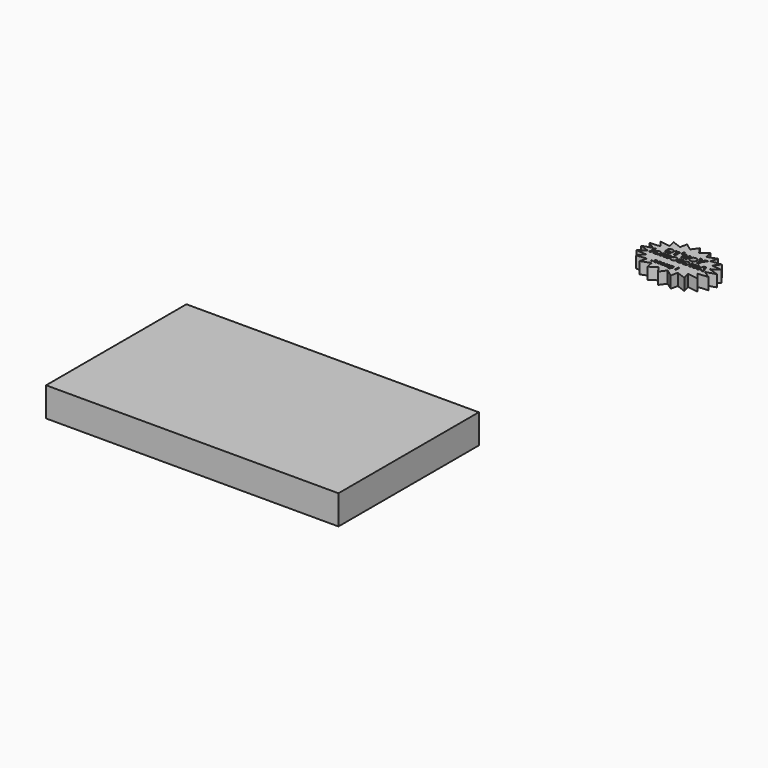
from build123d import *

# Parameters (mm, degrees)
F0_W     = 50
F0_H     = 30
F1_DEPTH = 5
F2_W     = 0.179312
F2_H     = 0.19276
F2_W_2   = 0.286899
F2_H_2   = 0.283711
F2_W_3   = 0.191765
F2_H_3   = 0.743647
F2_W_4   = 0.212485
F2_H_4   = 0.497591
F3_DEPTH = 2


# Not quite as in the source:
# - ends of sketch curves that miss each other by under 0.0002 mm in the source are joined


with BuildPart() as f1:
    # F0 (on Top) → F1 (new body)
    with BuildSketch(Plane.XY):
        with Locations((-4.7771148384, -0.2846198264)):
            Rectangle(F0_W, F0_H)
    extrude(amount=F1_DEPTH)


with BuildPart() as f3:
    # F2 (on Top) → F3 (new body)
    with BuildSketch(Plane.XY):
        Polygon((13.440635, 67.926958), (15.209908, 67.693765), (14.365041, 68.766458), (16.154706, 68.91293), (14.859046, 69.757273), (16.49392, 70.269073), (14.874297, 70.802416), (16.194345, 71.629444), (14.409299, 71.79958), (15.285305, 72.860881), (13.509569, 72.651155), (13.855785, 73.842842), (12.26318, 73.273785), (12.045715, 74.479207), (10.792136, 73.606521), (10.032278, 74.707683), (9.240434, 73.616793), (8.012563, 74.505905), (7.759965, 73.303595), (6.184273, 73.893626), (6.495648, 72.697586), (4.726375, 72.930778), (5.571243, 71.858085), (3.781577, 71.711613), (5.077236, 70.86727), (3.442363, 70.355471), (5.061986, 69.822128), (3.741938, 68.9951), (5.526984, 68.824963), (4.650977, 67.763662), (6.426714, 67.973388), (6.080498, 66.781701), (7.673103, 67.350759), (7.890568, 66.145336), (9.144147, 67.018023), (9.904005, 65.916861), (10.695849, 67.007751), (11.92372, 66.118638), (12.176318, 67.320948), (13.75201, 66.730918), align=None)
        with Locations((7.262146, 67.906265)):
            Rectangle(F2_W, F2_H, mode=Mode.SUBTRACT)
        with BuildLine():
            Line((7.542072, 68.214831), (7.542072, 68.350311))
            add(Edge.make_bspline(
                [(7.66012, 68.373721), (7.623925, 68.36874), (7.584576, 68.360937), (7.542072, 68.350311)],
                knots=[0, 0, 0, 0, 1, 1, 1, 1], degree=3))
            add(Edge.make_bspline(
                [(7.763722, 68.381192), (7.730848, 68.381192), (7.696314, 68.378702), (7.66012, 68.373721)],
                knots=[0, 0, 0, 0, 1, 1, 1, 1], degree=3))
            add(Edge.make_bspline(
                [(7.950008, 68.338357), (7.909496, 68.366913), (7.847401, 68.381192), (7.763722, 68.381192)],
                knots=[0, 0, 0, 0, 1, 1, 1, 1], degree=3))
            add(Edge.make_bspline(
                [(8.010775, 68.206861), (8.010775, 68.265968), (7.990519, 68.309799), (7.950008, 68.338357)],
                knots=[0, 0, 0, 0, 1, 1, 1, 1], degree=3))
            add(Edge.make_bspline(
                [(7.962958, 68.084331), (7.994836, 68.111228), (8.010775, 68.152071), (8.010775, 68.206861)],
                knots=[0, 0, 0, 0, 1, 1, 1, 1], degree=3))
            add(Edge.make_bspline(
                [(7.796098, 68.029043), (7.87546, 68.039005), (7.93108, 68.057434), (7.962958, 68.084331)],
                knots=[0, 0, 0, 0, 1, 1, 1, 1], degree=3))
            Line((7.796098, 68.029043), (7.764718, 68.02506))
            add(Edge.make_bspline(
                [(7.692495, 68.00663), (7.70445, 68.0146), (7.728524, 68.020743), (7.764718, 68.02506)],
                knots=[0, 0, 0, 0, 1, 1, 1, 1], degree=3))
            add(Edge.make_bspline(
                [(7.674066, 67.971266), (7.674066, 67.987205), (7.680209, 67.998993), (7.692495, 68.00663)],
                knots=[0, 0, 0, 0, 1, 1, 1, 1], degree=3))
            add(Edge.make_bspline(
                [(7.700465, 67.92843), (7.682866, 67.93806), (7.674066, 67.952339), (7.674066, 67.971266)],
                knots=[0, 0, 0, 0, 1, 1, 1, 1], degree=3))
            add(Edge.make_bspline(
                [(7.779163, 67.913986), (7.744297, 67.913986), (7.718064, 67.918801), (7.700465, 67.92843)],
                knots=[0, 0, 0, 0, 1, 1, 1, 1], degree=3))
            add(Edge.make_bspline(
                [(7.893226, 67.926936), (7.855703, 67.918303), (7.817682, 67.913986), (7.779163, 67.913986)],
                knots=[0, 0, 0, 0, 1, 1, 1, 1], degree=3))
            add(Edge.make_bspline(
                [(8.002307, 67.965787), (7.966777, 67.94852), (7.930416, 67.93557), (7.893226, 67.926936)],
                knots=[0, 0, 0, 0, 1, 1, 1, 1], degree=3))
            Line((8.002307, 67.965787), (8.002307, 67.830307))
            add(Edge.make_bspline(
                [(7.881271, 67.804406), (7.920454, 67.810051), (7.9608, 67.818685), (8.002307, 67.830307)],
                knots=[0, 0, 0, 0, 1, 1, 1, 1], degree=3))
            add(Edge.make_bspline(
                [(7.766711, 67.795441), (7.803569, 67.795441), (7.841756, 67.798429), (7.881271, 67.804406)],
                knots=[0, 0, 0, 0, 1, 1, 1, 1], degree=3))
            add(Edge.make_bspline(
                [(7.570464, 67.840269), (7.614295, 67.810383), (7.679711, 67.795441), (7.766711, 67.795441)],
                knots=[0, 0, 0, 0, 1, 1, 1, 1], degree=3))
            add(Edge.make_bspline(
                [(7.504716, 67.974255), (7.504716, 67.914816), (7.526632, 67.870154), (7.570464, 67.840269)],
                knots=[0, 0, 0, 0, 1, 1, 1, 1], degree=3))
            add(Edge.make_bspline(
                [(7.552034, 68.099275), (7.520489, 68.07271), (7.504716, 68.031037), (7.504716, 67.974255)],
                knots=[0, 0, 0, 0, 1, 1, 1, 1], degree=3))
            add(Edge.make_bspline(
                [(7.736327, 68.156555), (7.645011, 68.144933), (7.58358, 68.12584), (7.552034, 68.099275)],
                knots=[0, 0, 0, 0, 1, 1, 1, 1], degree=3))
            Line((7.736327, 68.156555), (7.767707, 68.161037))
            add(Edge.make_bspline(
                [(7.834949, 68.177973), (7.822331, 68.170335), (7.799917, 68.16469), (7.767707, 68.161037)],
                knots=[0, 0, 0, 0, 1, 1, 1, 1], degree=3))
            add(Edge.make_bspline(
                [(7.853378, 68.210846), (7.853378, 68.196568), (7.847235, 68.18561), (7.834949, 68.177973)],
                knots=[0, 0, 0, 0, 1, 1, 1, 1], degree=3))
            add(Edge.make_bspline(
                [(7.828972, 68.249697), (7.845243, 68.241396), (7.853378, 68.228446), (7.853378, 68.210846)],
                knots=[0, 0, 0, 0, 1, 1, 1, 1], degree=3))
            add(Edge.make_bspline(
                [(7.753262, 68.262648), (7.787132, 68.262648), (7.812369, 68.258331), (7.828972, 68.249697)],
                knots=[0, 0, 0, 0, 1, 1, 1, 1], degree=3))
            add(Edge.make_bspline(
                [(7.652648, 68.250693), (7.688179, 68.258663), (7.721717, 68.262648), (7.753262, 68.262648)],
                knots=[0, 0, 0, 0, 1, 1, 1, 1], degree=3))
            add(Edge.make_bspline(
                [(7.542072, 68.214831), (7.580259, 68.23077), (7.617118, 68.242724), (7.652648, 68.250693)],
                knots=[0, 0, 0, 0, 1, 1, 1, 1], degree=3))
        make_face(mode=Mode.SUBTRACT)
        with BuildLine():
            Line((8.149742, 68.214831), (8.149742, 68.350311))
            add(Edge.make_bspline(
                [(8.267789, 68.373721), (8.231594, 68.36874), (8.192245, 68.360937), (8.149742, 68.350311)],
                knots=[0, 0, 0, 0, 1, 1, 1, 1], degree=3))
            add(Edge.make_bspline(
                [(8.371391, 68.381192), (8.338517, 68.381192), (8.303983, 68.378702), (8.267789, 68.373721)],
                knots=[0, 0, 0, 0, 1, 1, 1, 1], degree=3))
            add(Edge.make_bspline(
                [(8.557677, 68.338357), (8.517165, 68.366913), (8.45507, 68.381192), (8.371391, 68.381192)],
                knots=[0, 0, 0, 0, 1, 1, 1, 1], degree=3))
            add(Edge.make_bspline(
                [(8.618444, 68.206861), (8.618444, 68.265968), (8.598188, 68.309799), (8.557677, 68.338357)],
                knots=[0, 0, 0, 0, 1, 1, 1, 1], degree=3))
            add(Edge.make_bspline(
                [(8.570627, 68.084331), (8.602505, 68.111228), (8.618444, 68.152071), (8.618444, 68.206861)],
                knots=[0, 0, 0, 0, 1, 1, 1, 1], degree=3))
            add(Edge.make_bspline(
                [(8.403767, 68.029043), (8.483129, 68.039005), (8.538749, 68.057434), (8.570627, 68.084331)],
                knots=[0, 0, 0, 0, 1, 1, 1, 1], degree=3))
            Line((8.403767, 68.029043), (8.372387, 68.02506))
            add(Edge.make_bspline(
                [(8.300164, 68.00663), (8.312119, 68.0146), (8.336193, 68.020743), (8.372387, 68.02506)],
                knots=[0, 0, 0, 0, 1, 1, 1, 1], degree=3))
            add(Edge.make_bspline(
                [(8.281735, 67.971266), (8.281735, 67.987205), (8.287878, 67.998993), (8.300164, 68.00663)],
                knots=[0, 0, 0, 0, 1, 1, 1, 1], degree=3))
            add(Edge.make_bspline(
                [(8.308134, 67.92843), (8.290535, 67.93806), (8.281735, 67.952339), (8.281735, 67.971266)],
                knots=[0, 0, 0, 0, 1, 1, 1, 1], degree=3))
            add(Edge.make_bspline(
                [(8.386832, 67.913986), (8.351966, 67.913986), (8.325733, 67.918801), (8.308134, 67.92843)],
                knots=[0, 0, 0, 0, 1, 1, 1, 1], degree=3))
            add(Edge.make_bspline(
                [(8.500894, 67.926936), (8.463372, 67.918303), (8.425351, 67.913986), (8.386832, 67.913986)],
                knots=[0, 0, 0, 0, 1, 1, 1, 1], degree=3))
            add(Edge.make_bspline(
                [(8.609976, 67.965787), (8.574446, 67.94852), (8.538085, 67.93557), (8.500894, 67.926936)],
                knots=[0, 0, 0, 0, 1, 1, 1, 1], degree=3))
            Line((8.609976, 67.965787), (8.609976, 67.830307))
            add(Edge.make_bspline(
                [(8.48894, 67.804406), (8.528123, 67.810051), (8.568469, 67.818685), (8.609976, 67.830307)],
                knots=[0, 0, 0, 0, 1, 1, 1, 1], degree=3))
            add(Edge.make_bspline(
                [(8.37438, 67.795441), (8.411238, 67.795441), (8.449425, 67.798429), (8.48894, 67.804406)],
                knots=[0, 0, 0, 0, 1, 1, 1, 1], degree=3))
            add(Edge.make_bspline(
                [(8.178133, 67.840269), (8.221964, 67.810383), (8.28738, 67.795441), (8.37438, 67.795441)],
                knots=[0, 0, 0, 0, 1, 1, 1, 1], degree=3))
            add(Edge.make_bspline(
                [(8.112385, 67.974255), (8.112385, 67.914816), (8.134301, 67.870154), (8.178133, 67.840269)],
                knots=[0, 0, 0, 0, 1, 1, 1, 1], degree=3))
            add(Edge.make_bspline(
                [(8.159703, 68.099275), (8.128158, 68.07271), (8.112385, 68.031037), (8.112385, 67.974255)],
                knots=[0, 0, 0, 0, 1, 1, 1, 1], degree=3))
            add(Edge.make_bspline(
                [(8.343996, 68.156555), (8.25268, 68.144933), (8.191249, 68.12584), (8.159703, 68.099275)],
                knots=[0, 0, 0, 0, 1, 1, 1, 1], degree=3))
            Line((8.343996, 68.156555), (8.375376, 68.161037))
            add(Edge.make_bspline(
                [(8.442618, 68.177973), (8.43, 68.170335), (8.407586, 68.16469), (8.375376, 68.161037)],
                knots=[0, 0, 0, 0, 1, 1, 1, 1], degree=3))
            add(Edge.make_bspline(
                [(8.461047, 68.210846), (8.461047, 68.196568), (8.454904, 68.18561), (8.442618, 68.177973)],
                knots=[0, 0, 0, 0, 1, 1, 1, 1], degree=3))
            add(Edge.make_bspline(
                [(8.436641, 68.249697), (8.452912, 68.241396), (8.461047, 68.228446), (8.461047, 68.210846)],
                knots=[0, 0, 0, 0, 1, 1, 1, 1], degree=3))
            add(Edge.make_bspline(
                [(8.360931, 68.262648), (8.394801, 68.262648), (8.420038, 68.258331), (8.436641, 68.249697)],
                knots=[0, 0, 0, 0, 1, 1, 1, 1], degree=3))
            add(Edge.make_bspline(
                [(8.260317, 68.250693), (8.295848, 68.258663), (8.329386, 68.262648), (8.360931, 68.262648)],
                knots=[0, 0, 0, 0, 1, 1, 1, 1], degree=3))
            add(Edge.make_bspline(
                [(8.149742, 68.214831), (8.187928, 68.23077), (8.224787, 68.242724), (8.260317, 68.250693)],
                knots=[0, 0, 0, 0, 1, 1, 1, 1], degree=3))
        make_face(mode=Mode.SUBTRACT)
        with BuildLine():
            Line((8.720054, 68.039503), (8.720054, 68.090309))
            add(Edge.make_bspline(
                [(8.79925, 68.301996), (8.746453, 68.249199), (8.720054, 68.178636), (8.720054, 68.090309)],
                knots=[0, 0, 0, 0, 1, 1, 1, 1], degree=3))
            add(Edge.make_bspline(
                [(9.009444, 68.381193), (8.92178, 68.381193), (8.851715, 68.354794), (8.79925, 68.301996)],
                knots=[0, 0, 0, 0, 1, 1, 1, 1], degree=3))
            add(Edge.make_bspline(
                [(9.236572, 68.302993), (9.181451, 68.355126), (9.105741, 68.381193), (9.009444, 68.381193)],
                knots=[0, 0, 0, 0, 1, 1, 1, 1], degree=3))
            add(Edge.make_bspline(
                [(9.318757, 68.088316), (9.318757, 68.1793), (9.291362, 68.250859), (9.236572, 68.302993)],
                knots=[0, 0, 0, 0, 1, 1, 1, 1], degree=3))
            add(Edge.make_bspline(
                [(9.235078, 67.872146), (9.290864, 67.923615), (9.318757, 67.995672), (9.318757, 68.088316)],
                knots=[0, 0, 0, 0, 1, 1, 1, 1], degree=3))
            add(Edge.make_bspline(
                [(8.999482, 67.79544), (9.100428, 67.79544), (9.17896, 67.821008), (9.235078, 67.872146)],
                knots=[0, 0, 0, 0, 1, 1, 1, 1], degree=3))
            add(Edge.make_bspline(
                [(8.872967, 67.807892), (8.915139, 67.79959), (8.95731, 67.79544), (8.999482, 67.79544)],
                knots=[0, 0, 0, 0, 1, 1, 1, 1], degree=3))
            add(Edge.make_bspline(
                [(8.746453, 67.843755), (8.788624, 67.827816), (8.830796, 67.815861), (8.872967, 67.807892)],
                knots=[0, 0, 0, 0, 1, 1, 1, 1], degree=3))
            Line((8.746453, 67.843755), (8.746453, 67.981227))
            add(Edge.make_bspline(
                [(8.867986, 67.930422), (8.828471, 67.941712), (8.78796, 67.958647), (8.746453, 67.981227)],
                knots=[0, 0, 0, 0, 1, 1, 1, 1], degree=3))
            add(Edge.make_bspline(
                [(8.983045, 67.913985), (8.945522, 67.913985), (8.907169, 67.919464), (8.867986, 67.930422)],
                knots=[0, 0, 0, 0, 1, 1, 1, 1], degree=3))
            add(Edge.make_bspline(
                [(9.091629, 67.945365), (9.065728, 67.924445), (9.029533, 67.913985), (8.983045, 67.913985)],
                knots=[0, 0, 0, 0, 1, 1, 1, 1], degree=3))
            add(Edge.make_bspline(
                [(9.136955, 68.039503), (9.132638, 67.997664), (9.117529, 67.966285), (9.091629, 67.945365)],
                knots=[0, 0, 0, 0, 1, 1, 1, 1], degree=3))
            Line((9.136955, 68.039503), (8.720054, 68.039503))
        make_face(mode=Mode.SUBTRACT)
        with BuildLine():
            Line((10.010105, 68.367745), (10.010105, 68.027051))
            add(Edge.make_bspline(
                [(9.9598, 67.854712), (9.993338, 67.894228), (10.010107, 67.951674), (10.010105, 68.027051)],
                knots=[0, 0, 0, 0, 1, 1, 1, 1], degree=3))
            add(Edge.make_bspline(
                [(9.812365, 67.79544), (9.876785, 67.79544), (9.92593, 67.815197), (9.9598, 67.854712)],
                knots=[0, 0, 0, 0, 1, 1, 1, 1], degree=3))
            add(Edge.make_bspline(
                [(9.713245, 67.818352), (9.743131, 67.803077), (9.776171, 67.79544), (9.812365, 67.79544)],
                knots=[0, 0, 0, 0, 1, 1, 1, 1], degree=3))
            add(Edge.make_bspline(
                [(9.627574, 67.890575), (9.654471, 67.858033), (9.683028, 67.833959), (9.713245, 67.818352)],
                knots=[0, 0, 0, 0, 1, 1, 1, 1], degree=3))
            Line((9.627574, 67.890575), (9.627574, 67.809885))
            Line((9.627574, 67.809885), (9.449258, 67.809885))
            Line((9.449258, 67.809885), (9.449258, 68.367745))
            Line((9.449258, 68.367745), (9.627574, 68.367745))
            Line((9.627574, 68.367745), (9.627574, 68.092301))
            add(Edge.make_bspline(
                [(9.659452, 67.973258), (9.6382, 68.001815), (9.627574, 68.041496), (9.627574, 68.092301)],
                knots=[0, 0, 0, 0, 1, 1, 1, 1], degree=3))
            add(Edge.make_bspline(
                [(9.747116, 67.930422), (9.709925, 67.930422), (9.680704, 67.944701), (9.659452, 67.973258)],
                knots=[0, 0, 0, 0, 1, 1, 1, 1], degree=3))
            add(Edge.make_bspline(
                [(9.787959, 67.939886), (9.776005, 67.933577), (9.76239, 67.930422), (9.747116, 67.930422)],
                knots=[0, 0, 0, 0, 1, 1, 1, 1], degree=3))
            add(Edge.make_bspline(
                [(9.81635, 67.966783), (9.809045, 67.955161), (9.799581, 67.946195), (9.787959, 67.939886)],
                knots=[0, 0, 0, 0, 1, 1, 1, 1], degree=3))
            add(Edge.make_bspline(
                [(9.828304, 68.009618), (9.82598, 67.990027), (9.821995, 67.975748), (9.81635, 67.966783)],
                knots=[0, 0, 0, 0, 1, 1, 1, 1], degree=3))
            add(Edge.make_bspline(
                [(9.831791, 68.106746), (9.831791, 68.061918), (9.830629, 68.029542), (9.828304, 68.009618)],
                knots=[0, 0, 0, 0, 1, 1, 1, 1], degree=3))
            add(Edge.make_bspline(
                [(9.831292, 68.197896), (9.831624, 68.152404), (9.831791, 68.122021), (9.831791, 68.106746)],
                knots=[0, 0, 0, 0, 1, 1, 1, 1], degree=3))
            add(Edge.make_bspline(
                [(9.830793, 68.311959), (9.830793, 68.281741), (9.830959, 68.24372), (9.831292, 68.197896)],
                knots=[0, 0, 0, 0, 1, 1, 1, 1], degree=3))
            Line((9.830793, 68.311959), (9.830793, 68.367745))
            Line((9.830793, 68.367745), (10.010105, 68.367745))
        make_face(mode=Mode.SUBTRACT)
        with Locations((5.4750865, 69.8638915)):
            Rectangle(F2_W_2, F2_H_2, mode=Mode.SUBTRACT)
        with BuildLine():
            Line((5.925359, 70.089427), (5.925359, 70.170715))
            add(Edge.make_bspline(
                [(6.052073, 70.509416), (5.967597, 70.42494), (5.925359, 70.31204), (5.925359, 70.170715)],
                knots=[0, 0, 0, 0, 1, 1, 1, 1], degree=3))
            add(Edge.make_bspline(
                [(6.388383, 70.63613), (6.248121, 70.63613), (6.136018, 70.593892), (6.052073, 70.509416)],
                knots=[0, 0, 0, 0, 1, 1, 1, 1], degree=3))
            add(Edge.make_bspline(
                [(6.751789, 70.51101), (6.663594, 70.594423), (6.542459, 70.63613), (6.388383, 70.63613)],
                knots=[0, 0, 0, 0, 1, 1, 1, 1], degree=3))
            add(Edge.make_bspline(
                [(6.883285, 70.167527), (6.883285, 70.313102), (6.839453, 70.427596), (6.751789, 70.51101)],
                knots=[0, 0, 0, 0, 1, 1, 1, 1], degree=3))
            add(Edge.make_bspline(
                [(6.749398, 69.821654), (6.838656, 69.904005), (6.883285, 70.019296), (6.883285, 70.167527)],
                knots=[0, 0, 0, 0, 1, 1, 1, 1], degree=3))
            add(Edge.make_bspline(
                [(6.372444, 69.698925), (6.533958, 69.698925), (6.659609, 69.739835), (6.749398, 69.821654)],
                knots=[0, 0, 0, 0, 1, 1, 1, 1], degree=3))
            add(Edge.make_bspline(
                [(6.170021, 69.718848), (6.237495, 69.705566), (6.30497, 69.698925), (6.372444, 69.698925)],
                knots=[0, 0, 0, 0, 1, 1, 1, 1], degree=3))
            add(Edge.make_bspline(
                [(5.967597, 69.776228), (6.035072, 69.750726), (6.102546, 69.731599), (6.170021, 69.718848)],
                knots=[0, 0, 0, 0, 1, 1, 1, 1], degree=3))
            Line((5.967597, 69.776228), (5.967597, 69.996184))
            add(Edge.make_bspline(
                [(6.162051, 69.914896), (6.098827, 69.93296), (6.034009, 69.960056), (5.967597, 69.996184)],
                knots=[0, 0, 0, 0, 1, 1, 1, 1], degree=3))
            add(Edge.make_bspline(
                [(6.346145, 69.888597), (6.286109, 69.888597), (6.224744, 69.897363), (6.162051, 69.914896)],
                knots=[0, 0, 0, 0, 1, 1, 1, 1], degree=3))
            add(Edge.make_bspline(
                [(6.519879, 69.938804), (6.478438, 69.905333), (6.420526, 69.888597), (6.346145, 69.888597)],
                knots=[0, 0, 0, 0, 1, 1, 1, 1], degree=3))
            add(Edge.make_bspline(
                [(6.592401, 70.089427), (6.585494, 70.022483), (6.56132, 69.972276), (6.519879, 69.938804)],
                knots=[0, 0, 0, 0, 1, 1, 1, 1], degree=3))
            Line((6.592401, 70.089427), (5.925359, 70.089427))
        make_face(mode=Mode.SUBTRACT)
        with BuildLine():
            add(Edge.make_bspline(
                [(7.691385, 70.466381), (7.655257, 70.521636), (7.612487, 70.563608), (7.563077, 70.592298)],
                knots=[0, 0, 0, 0, 1, 1, 1, 1], degree=3))
            add(Edge.make_bspline(
                [(7.798972, 70.591501), (7.751687, 70.561748), (7.715825, 70.520042), (7.691385, 70.466381)],
                knots=[0, 0, 0, 0, 1, 1, 1, 1], degree=3))
            add(Edge.make_bspline(
                [(7.962346, 70.63613), (7.900716, 70.63613), (7.846258, 70.621253), (7.798972, 70.591501)],
                knots=[0, 0, 0, 0, 1, 1, 1, 1], degree=3))
            add(Edge.make_bspline(
                [(8.112968, 70.597876), (8.067277, 70.623379), (8.017069, 70.63613), (7.962346, 70.63613)],
                knots=[0, 0, 0, 0, 1, 1, 1, 1], degree=3))
            add(Edge.make_bspline(
                [(8.233306, 70.483914), (8.198241, 70.534387), (8.158128, 70.572374), (8.112968, 70.597876)],
                knots=[0, 0, 0, 0, 1, 1, 1, 1], degree=3))
            Line((8.233306, 70.483914), (8.233306, 70.614612))
            Line((8.233306, 70.614612), (8.520206, 70.614612))
            Line((8.520206, 70.614612), (8.520206, 69.722036))
            Line((8.520206, 69.722036), (8.233306, 69.722036))
            Line((8.233306, 69.722036), (8.233306, 70.161151))
            add(Edge.make_bspline(
                [(8.188678, 70.353215), (8.21843, 70.308586), (8.233306, 70.244565), (8.233306, 70.161151)],
                knots=[0, 0, 0, 0, 1, 1, 1, 1], degree=3))
            add(Edge.make_bspline(
                [(8.061964, 70.420955), (8.116687, 70.420955), (8.158925, 70.398375), (8.188678, 70.353215)],
                knots=[0, 0, 0, 0, 1, 1, 1, 1], degree=3))
            add(Edge.make_bspline(
                [(7.971112, 70.37792), (7.988114, 70.40661), (8.018397, 70.420955), (8.061964, 70.420955)],
                knots=[0, 0, 0, 0, 1, 1, 1, 1], degree=3))
            add(Edge.make_bspline(
                [(7.94561, 70.187451), (7.94561, 70.286272), (7.954111, 70.349761), (7.971112, 70.37792)],
                knots=[0, 0, 0, 0, 1, 1, 1, 1], degree=3))
            Line((7.94561, 70.187451), (7.94561, 69.722036))
            Line((7.94561, 69.722036), (7.658711, 69.722036))
            Line((7.658711, 69.722036), (7.658711, 70.160355))
            add(Edge.make_bspline(
                [(7.613285, 70.354012), (7.642506, 70.309383), (7.657648, 70.244831), (7.658711, 70.160355)],
                knots=[0, 0, 0, 0, 1, 1, 1, 1], degree=3))
            add(Edge.make_bspline(
                [(7.487368, 70.420955), (7.54156, 70.420955), (7.583532, 70.398641), (7.613285, 70.354012)],
                knots=[0, 0, 0, 0, 1, 1, 1, 1], degree=3))
            add(Edge.make_bspline(
                [(7.397313, 70.37792), (7.415909, 70.40661), (7.445927, 70.420955), (7.487368, 70.420955)],
                knots=[0, 0, 0, 0, 1, 1, 1, 1], degree=3))
            add(Edge.make_bspline(
                [(7.36942, 70.240846), (7.36942, 70.30407), (7.378718, 70.349761), (7.397313, 70.37792)],
                knots=[0, 0, 0, 0, 1, 1, 1, 1], degree=3))
            add(Edge.make_bspline(
                [(7.370217, 70.208968), (7.369686, 70.216406), (7.36942, 70.227032), (7.36942, 70.240846)],
                knots=[0, 0, 0, 0, 1, 1, 1, 1], degree=3))
            add(Edge.make_bspline(
                [(7.371014, 70.187451), (7.370482, 70.194358), (7.370217, 70.20153), (7.370217, 70.208968)],
                knots=[0, 0, 0, 0, 1, 1, 1, 1], degree=3))
            Line((7.371014, 70.187451), (7.371014, 69.722036))
            Line((7.371014, 69.722036), (7.084114, 69.722036))
            Line((7.084114, 69.722036), (7.084114, 70.265551))
            add(Edge.make_bspline(
                [(7.164605, 70.541293), (7.110944, 70.478069), (7.084114, 70.386155), (7.084114, 70.265551)],
                knots=[0, 0, 0, 0, 1, 1, 1, 1], degree=3))
            add(Edge.make_bspline(
                [(7.398907, 70.63613), (7.296367, 70.63613), (7.218266, 70.604518), (7.164605, 70.541293)],
                knots=[0, 0, 0, 0, 1, 1, 1, 1], degree=3))
            add(Edge.make_bspline(
                [(7.563077, 70.592298), (7.513135, 70.621519), (7.458412, 70.63613), (7.398907, 70.63613)],
                knots=[0, 0, 0, 0, 1, 1, 1, 1], degree=3))
        make_face(mode=Mode.SUBTRACT)
        with BuildLine():
            add(Edge.make_bspline(
                [(9.215937, 70.63613), (9.062392, 70.63613), (8.942585, 70.594689), (8.856515, 70.511807)],
                knots=[0, 0, 0, 0, 1, 1, 1, 1], degree=3))
            add(Edge.make_bspline(
                [(9.577749, 70.511807), (9.490616, 70.594689), (9.370012, 70.63613), (9.215937, 70.63613)],
                knots=[0, 0, 0, 0, 1, 1, 1, 1], degree=3))
            add(Edge.make_bspline(
                [(9.707651, 70.167527), (9.707651, 70.314165), (9.66435, 70.428924), (9.577749, 70.511807)],
                knots=[0, 0, 0, 0, 1, 1, 1, 1], degree=3))
            add(Edge.make_bspline(
                [(9.577749, 69.823248), (9.66435, 69.90613), (9.707651, 70.02089), (9.707651, 70.167527)],
                knots=[0, 0, 0, 0, 1, 1, 1, 1], degree=3))
            add(Edge.make_bspline(
                [(9.215937, 69.698925), (9.370012, 69.698925), (9.490616, 69.740366), (9.577749, 69.823248)],
                knots=[0, 0, 0, 0, 1, 1, 1, 1], degree=3))
            add(Edge.make_bspline(
                [(8.856515, 69.823248), (8.942585, 69.740366), (9.062392, 69.698925), (9.215937, 69.698925)],
                knots=[0, 0, 0, 0, 1, 1, 1, 1], degree=3))
            add(Edge.make_bspline(
                [(8.726614, 70.167527), (8.726614, 70.02089), (8.769914, 69.90613), (8.856515, 69.823248)],
                knots=[0, 0, 0, 0, 1, 1, 1, 1], degree=3))
            add(Edge.make_bspline(
                [(8.856515, 70.511807), (8.769914, 70.428924), (8.726614, 70.314165), (8.726614, 70.167527)],
                knots=[0, 0, 0, 0, 1, 1, 1, 1], degree=3))
        make_face(mode=Mode.SUBTRACT)
        with BuildLine():
            add(Edge.make_bspline(
                [(10.355779, 67.904521), (10.380352, 67.871979), (10.407415, 67.848071), (10.436968, 67.832796)],
                knots=[0, 0, 0, 0, 1, 1, 1, 1], degree=3))
            Line((10.355779, 67.904521), (10.355779, 67.866169))
            add(Edge.make_bspline(
                [(10.396623, 67.746129), (10.369394, 67.771698), (10.355779, 67.811711), (10.355779, 67.866169)],
                knots=[0, 0, 0, 0, 1, 1, 1, 1], degree=3))
            add(Edge.make_bspline(
                [(10.52513, 67.707776), (10.466687, 67.707776), (10.423851, 67.720561), (10.396623, 67.746129)],
                knots=[0, 0, 0, 0, 1, 1, 1, 1], degree=3))
            add(Edge.make_bspline(
                [(10.615284, 67.721224), (10.585399, 67.712259), (10.555347, 67.707776), (10.52513, 67.707776)],
                knots=[0, 0, 0, 0, 1, 1, 1, 1], degree=3))
            add(Edge.make_bspline(
                [(10.706932, 67.761072), (10.675719, 67.743141), (10.645169, 67.729858), (10.615284, 67.721224)],
                knots=[0, 0, 0, 0, 1, 1, 1, 1], degree=3))
            Line((10.706932, 67.761072), (10.706932, 67.622104))
            add(Edge.make_bspline(
                [(10.608809, 67.597698), (10.641351, 67.603011), (10.674059, 67.611147), (10.706932, 67.622104)],
                knots=[0, 0, 0, 0, 1, 1, 1, 1], degree=3))
            add(Edge.make_bspline(
                [(10.507696, 67.589729), (10.542563, 67.589729), (10.576267, 67.592385), (10.608809, 67.597698)],
                knots=[0, 0, 0, 0, 1, 1, 1, 1], degree=3))
            add(Edge.make_bspline(
                [(10.261641, 67.660956), (10.318091, 67.613471), (10.400109, 67.589729), (10.507696, 67.589729)],
                knots=[0, 0, 0, 0, 1, 1, 1, 1], degree=3))
            add(Edge.make_bspline(
                [(10.176467, 67.866169), (10.176467, 67.776513), (10.204858, 67.708108), (10.261641, 67.660956)],
                knots=[0, 0, 0, 0, 1, 1, 1, 1], degree=3))
            Line((10.176467, 67.866169), (10.176467, 68.367745))
            Line((10.176467, 68.367745), (10.355779, 68.367745))
            Line((10.355779, 68.367745), (10.355779, 68.285062))
            add(Edge.make_bspline(
                [(10.436968, 68.357285), (10.407415, 68.34201), (10.380352, 68.317936), (10.355779, 68.285062)],
                knots=[0, 0, 0, 0, 1, 1, 1, 1], degree=3))
            add(Edge.make_bspline(
                [(10.539574, 68.380196), (10.500723, 68.380196), (10.466521, 68.372559), (10.436968, 68.357285)],
                knots=[0, 0, 0, 0, 1, 1, 1, 1], degree=3))
            add(Edge.make_bspline(
                [(10.708427, 68.300004), (10.663931, 68.353466), (10.607646, 68.380196), (10.539574, 68.380196)],
                knots=[0, 0, 0, 0, 1, 1, 1, 1], degree=3))
            add(Edge.make_bspline(
                [(10.77517, 68.095289), (10.77517, 68.178636), (10.752922, 68.246875), (10.708427, 68.300004)],
                knots=[0, 0, 0, 0, 1, 1, 1, 1], degree=3))
            add(Edge.make_bspline(
                [(10.708427, 67.890077), (10.752922, 67.943871), (10.77517, 68.012275), (10.77517, 68.095289)],
                knots=[0, 0, 0, 0, 1, 1, 1, 1], degree=3))
            add(Edge.make_bspline(
                [(10.539574, 67.809885), (10.607646, 67.809885), (10.663931, 67.836616), (10.708427, 67.890077)],
                knots=[0, 0, 0, 0, 1, 1, 1, 1], degree=3))
            add(Edge.make_bspline(
                [(10.436968, 67.832796), (10.466521, 67.817522), (10.500723, 67.809885), (10.539574, 67.809885)],
                knots=[0, 0, 0, 0, 1, 1, 1, 1], degree=3))
        make_face(mode=Mode.SUBTRACT)
        with Locations((11.3666515, 68.1817085)):
            Rectangle(F2_W_3, F2_H_3, mode=Mode.SUBTRACT)
        with BuildLine():
            Line((9.915653, 70.369951), (9.915653, 70.586719))
            add(Edge.make_bspline(
                [(10.104529, 70.624175), (10.046617, 70.616206), (9.983659, 70.603721), (9.915653, 70.586719)],
                knots=[0, 0, 0, 0, 1, 1, 1, 1], degree=3))
            add(Edge.make_bspline(
                [(10.270292, 70.63613), (10.217694, 70.63613), (10.16244, 70.632145), (10.104529, 70.624175)],
                knots=[0, 0, 0, 0, 1, 1, 1, 1], degree=3))
            add(Edge.make_bspline(
                [(10.568349, 70.567592), (10.503531, 70.613284), (10.404179, 70.63613), (10.270292, 70.63613)],
                knots=[0, 0, 0, 0, 1, 1, 1, 1], degree=3))
            add(Edge.make_bspline(
                [(10.665576, 70.3572), (10.665576, 70.45177), (10.633167, 70.521901), (10.568349, 70.567592)],
                knots=[0, 0, 0, 0, 1, 1, 1, 1], degree=3))
            add(Edge.make_bspline(
                [(10.589069, 70.161151), (10.640074, 70.204186), (10.665576, 70.269536), (10.665576, 70.3572)],
                knots=[0, 0, 0, 0, 1, 1, 1, 1], degree=3))
            add(Edge.make_bspline(
                [(10.322094, 70.072691), (10.449073, 70.08863), (10.538065, 70.118116), (10.589069, 70.161151)],
                knots=[0, 0, 0, 0, 1, 1, 1, 1], degree=3))
            Line((10.322094, 70.072691), (10.271886, 70.066315))
            add(Edge.make_bspline(
                [(10.15633, 70.036828), (10.175456, 70.04958), (10.213975, 70.059409), (10.271886, 70.066315)],
                knots=[0, 0, 0, 0, 1, 1, 1, 1], degree=3))
            add(Edge.make_bspline(
                [(10.126843, 69.980246), (10.126843, 70.005748), (10.136672, 70.024608), (10.15633, 70.036828)],
                knots=[0, 0, 0, 0, 1, 1, 1, 1], degree=3))
            add(Edge.make_bspline(
                [(10.169081, 69.911709), (10.140922, 69.927116), (10.126843, 69.949962), (10.126843, 69.980246)],
                knots=[0, 0, 0, 0, 1, 1, 1, 1], degree=3))
            add(Edge.make_bspline(
                [(10.294998, 69.888597), (10.239212, 69.888597), (10.197239, 69.896301), (10.169081, 69.911709)],
                knots=[0, 0, 0, 0, 1, 1, 1, 1], degree=3))
            add(Edge.make_bspline(
                [(10.477497, 69.909317), (10.417461, 69.895504), (10.356628, 69.888597), (10.294998, 69.888597)],
                knots=[0, 0, 0, 0, 1, 1, 1, 1], degree=3))
            add(Edge.make_bspline(
                [(10.652028, 69.971479), (10.595179, 69.943852), (10.537002, 69.923131), (10.477497, 69.909317)],
                knots=[0, 0, 0, 0, 1, 1, 1, 1], degree=3))
            Line((10.652028, 69.971479), (10.652028, 69.754711))
            add(Edge.make_bspline(
                [(10.458371, 69.713269), (10.521064, 69.722302), (10.585616, 69.736115), (10.652028, 69.754711)],
                knots=[0, 0, 0, 0, 1, 1, 1, 1], degree=3))
            add(Edge.make_bspline(
                [(10.275074, 69.698925), (10.334048, 69.698925), (10.395147, 69.703706), (10.458371, 69.713269)],
                knots=[0, 0, 0, 0, 1, 1, 1, 1], degree=3))
            add(Edge.make_bspline(
                [(9.961078, 69.770649), (10.03121, 69.722833), (10.135875, 69.698925), (10.275074, 69.698925)],
                knots=[0, 0, 0, 0, 1, 1, 1, 1], degree=3))
            add(Edge.make_bspline(
                [(9.855882, 69.985027), (9.855882, 69.889925), (9.890948, 69.818466), (9.961078, 69.770649)],
                knots=[0, 0, 0, 0, 1, 1, 1, 1], degree=3))
            add(Edge.make_bspline(
                [(9.931592, 70.18506), (9.881119, 70.142556), (9.855882, 70.075879), (9.855882, 69.985027)],
                knots=[0, 0, 0, 0, 1, 1, 1, 1], degree=3))
            add(Edge.make_bspline(
                [(10.226461, 70.276708), (10.080354, 70.258113), (9.982065, 70.227563), (9.931592, 70.18506)],
                knots=[0, 0, 0, 0, 1, 1, 1, 1], degree=3))
            Line((10.226461, 70.276708), (10.276668, 70.283881))
            add(Edge.make_bspline(
                [(10.384255, 70.310977), (10.364066, 70.298757), (10.328203, 70.289725), (10.276668, 70.283881)],
                knots=[0, 0, 0, 0, 1, 1, 1, 1], degree=3))
            add(Edge.make_bspline(
                [(10.413742, 70.363575), (10.413742, 70.340729), (10.403913, 70.323197), (10.384255, 70.310977)],
                knots=[0, 0, 0, 0, 1, 1, 1, 1], degree=3))
            add(Edge.make_bspline(
                [(10.374692, 70.425737), (10.400726, 70.412454), (10.413742, 70.391734), (10.413742, 70.363575)],
                knots=[0, 0, 0, 0, 1, 1, 1, 1], degree=3))
            add(Edge.make_bspline(
                [(10.253556, 70.446457), (10.307749, 70.446457), (10.348127, 70.43955), (10.374692, 70.425737)],
                knots=[0, 0, 0, 0, 1, 1, 1, 1], degree=3))
            add(Edge.make_bspline(
                [(10.092574, 70.427331), (10.149423, 70.440082), (10.203083, 70.446457), (10.253556, 70.446457)],
                knots=[0, 0, 0, 0, 1, 1, 1, 1], degree=3))
            add(Edge.make_bspline(
                [(9.915653, 70.369951), (9.976752, 70.395453), (10.035725, 70.414579), (10.092574, 70.427331)],
                knots=[0, 0, 0, 0, 1, 1, 1, 1], degree=3))
        make_face(mode=Mode.SUBTRACT)
        with BuildLine():
            Line((10.828152, 70.089427), (10.828152, 70.170715))
            add(Edge.make_bspline(
                [(10.954866, 70.509416), (10.87039, 70.42494), (10.828152, 70.31204), (10.828152, 70.170715)],
                knots=[0, 0, 0, 0, 1, 1, 1, 1], degree=3))
            add(Edge.make_bspline(
                [(11.291177, 70.63613), (11.150914, 70.63613), (11.038811, 70.593892), (10.954866, 70.509416)],
                knots=[0, 0, 0, 0, 1, 1, 1, 1], degree=3))
            add(Edge.make_bspline(
                [(11.654582, 70.51101), (11.566387, 70.594423), (11.445252, 70.63613), (11.291177, 70.63613)],
                knots=[0, 0, 0, 0, 1, 1, 1, 1], degree=3))
            add(Edge.make_bspline(
                [(11.786078, 70.167527), (11.786078, 70.313102), (11.742246, 70.427596), (11.654582, 70.51101)],
                knots=[0, 0, 0, 0, 1, 1, 1, 1], degree=3))
            add(Edge.make_bspline(
                [(11.652192, 69.821654), (11.741449, 69.904005), (11.786078, 70.019296), (11.786078, 70.167527)],
                knots=[0, 0, 0, 0, 1, 1, 1, 1], degree=3))
            add(Edge.make_bspline(
                [(11.275237, 69.698925), (11.436751, 69.698925), (11.562403, 69.739835), (11.652192, 69.821654)],
                knots=[0, 0, 0, 0, 1, 1, 1, 1], degree=3))
            add(Edge.make_bspline(
                [(11.072814, 69.718848), (11.140288, 69.705566), (11.207763, 69.698925), (11.275237, 69.698925)],
                knots=[0, 0, 0, 0, 1, 1, 1, 1], degree=3))
            add(Edge.make_bspline(
                [(10.87039, 69.776228), (10.937865, 69.750726), (11.00534, 69.731599), (11.072814, 69.718848)],
                knots=[0, 0, 0, 0, 1, 1, 1, 1], degree=3))
            Line((10.87039, 69.776228), (10.87039, 69.996184))
            add(Edge.make_bspline(
                [(11.064844, 69.914896), (11.00162, 69.93296), (10.936802, 69.960056), (10.87039, 69.996184)],
                knots=[0, 0, 0, 0, 1, 1, 1, 1], degree=3))
            add(Edge.make_bspline(
                [(11.248938, 69.888597), (11.188902, 69.888597), (11.127537, 69.897363), (11.064844, 69.914896)],
                knots=[0, 0, 0, 0, 1, 1, 1, 1], degree=3))
            add(Edge.make_bspline(
                [(11.422672, 69.938804), (11.381231, 69.905333), (11.32332, 69.888597), (11.248938, 69.888597)],
                knots=[0, 0, 0, 0, 1, 1, 1, 1], degree=3))
            add(Edge.make_bspline(
                [(11.495194, 70.089427), (11.488287, 70.022483), (11.464113, 69.972276), (11.422672, 69.938804)],
                knots=[0, 0, 0, 0, 1, 1, 1, 1], degree=3))
            Line((11.495194, 70.089427), (10.828152, 70.089427))
        make_face(mode=Mode.SUBTRACT)
        Polygon((13.029309, 70.614612), (13.306646, 70.614612), (13.071547, 69.722036), (12.759942, 69.722036), (12.610117, 70.335682), (12.459495, 69.722036), (12.14789, 69.722036), (11.912792, 70.614612), (12.190129, 70.614612), (12.34075, 70.005747), (12.490576, 70.614612), (12.728862, 70.614612), (12.879484, 69.999372), align=None, mode=Mode.SUBTRACT)
        Polygon((5.331637, 70.911872), (5.618536, 70.911872), (5.618536, 70.455224), (5.577892, 70.122101), (5.372281, 70.122101), (5.331637, 70.455224), align=None, mode=Mode.SUBTRACT)
        with BuildLine():
            Line((6.865965, 71.502052), (6.865965, 71.593501))
            add(Edge.make_bspline(
                [(7.008519, 71.974539), (6.913483, 71.879504), (6.865965, 71.752491), (6.865965, 71.593501)],
                knots=[0, 0, 0, 0, 1, 1, 1, 1], degree=3))
            add(Edge.make_bspline(
                [(7.386867, 72.117092), (7.229072, 72.117092), (7.102956, 72.069575), (7.008519, 71.974539)],
                knots=[0, 0, 0, 0, 1, 1, 1, 1], degree=3))
            add(Edge.make_bspline(
                [(7.795699, 71.976332), (7.69648, 72.070172), (7.560202, 72.117092), (7.386867, 72.117092)],
                knots=[0, 0, 0, 0, 1, 1, 1, 1], degree=3))
            add(Edge.make_bspline(
                [(7.943631, 71.589915), (7.943631, 71.753686), (7.894321, 71.882492), (7.795699, 71.976332)],
                knots=[0, 0, 0, 0, 1, 1, 1, 1], degree=3))
            add(Edge.make_bspline(
                [(7.793009, 71.200807), (7.893424, 71.293452), (7.943631, 71.423154), (7.943631, 71.589915)],
                knots=[0, 0, 0, 0, 1, 1, 1, 1], degree=3))
            add(Edge.make_bspline(
                [(7.368936, 71.062737), (7.550639, 71.062737), (7.691997, 71.10876), (7.793009, 71.200807)],
                knots=[0, 0, 0, 0, 1, 1, 1, 1], degree=3))
            add(Edge.make_bspline(
                [(7.14121, 71.085151), (7.217118, 71.070208), (7.293027, 71.062737), (7.368936, 71.062737)],
                knots=[0, 0, 0, 0, 1, 1, 1, 1], degree=3))
            add(Edge.make_bspline(
                [(6.913483, 71.149703), (6.989392, 71.121013), (7.065301, 71.099496), (7.14121, 71.085151)],
                knots=[0, 0, 0, 0, 1, 1, 1, 1], degree=3))
            Line((6.913483, 71.149703), (6.913483, 71.397154))
            add(Edge.make_bspline(
                [(7.132244, 71.305705), (7.061117, 71.326027), (6.988196, 71.35651), (6.913483, 71.397154)],
                knots=[0, 0, 0, 0, 1, 1, 1, 1], degree=3))
            add(Edge.make_bspline(
                [(7.33935, 71.276118), (7.271809, 71.276118), (7.202773, 71.28598), (7.132244, 71.305705)],
                knots=[0, 0, 0, 0, 1, 1, 1, 1], degree=3))
            add(Edge.make_bspline(
                [(7.5348, 71.332602), (7.488179, 71.294946), (7.423029, 71.276118), (7.33935, 71.276118)],
                knots=[0, 0, 0, 0, 1, 1, 1, 1], degree=3))
            add(Edge.make_bspline(
                [(7.616387, 71.502052), (7.608617, 71.42674), (7.581421, 71.370257), (7.5348, 71.332602)],
                knots=[0, 0, 0, 0, 1, 1, 1, 1], degree=3))
            Line((7.616387, 71.502052), (6.865965, 71.502052))
        make_face(mode=Mode.SUBTRACT)
        with BuildLine():
            add(Edge.make_bspline(
                [(8.029701, 71.819434), (8.057793, 71.832584), (8.085886, 71.842147), (8.113978, 71.848124)],
                knots=[0, 0, 0, 0, 1, 1, 1, 1], degree=3))
            Line((8.029701, 71.819434), (8.030598, 72.10992))
            add(Edge.make_bspline(
                [(8.085288, 72.115299), (8.072736, 72.114701), (8.054506, 72.112908), (8.030598, 72.10992)],
                knots=[0, 0, 0, 0, 1, 1, 1, 1], degree=3))
            add(Edge.make_bspline(
                [(8.120254, 72.117092), (8.109495, 72.117092), (8.09784, 72.116495), (8.085288, 72.115299)],
                knots=[0, 0, 0, 0, 1, 1, 1, 1], degree=3))
            add(Edge.make_bspline(
                [(8.313014, 72.071368), (8.259221, 72.101851), (8.194967, 72.117092), (8.120254, 72.117092)],
                knots=[0, 0, 0, 0, 1, 1, 1, 1], degree=3))
            add(Edge.make_bspline(
                [(8.454671, 71.927918), (8.413429, 71.993666), (8.36621, 72.041482), (8.313014, 72.071368)],
                knots=[0, 0, 0, 0, 1, 1, 1, 1], degree=3))
            Line((8.454671, 71.927918), (8.454671, 72.092885))
            Line((8.454671, 72.092885), (8.77564, 72.092885))
            Line((8.77564, 72.092885), (8.77564, 71.088737))
            Line((8.77564, 71.088737), (8.454671, 71.088737))
            Line((8.454671, 71.088737), (8.454671, 71.551362))
            add(Edge.make_bspline(
                [(8.388326, 71.778192), (8.432556, 71.725594), (8.454671, 71.649984), (8.454671, 71.551362)],
                knots=[0, 0, 0, 0, 1, 1, 1, 1], degree=3))
            add(Edge.make_bspline(
                [(8.197358, 71.857986), (8.279842, 71.857986), (8.343498, 71.831388), (8.388326, 71.778192)],
                knots=[0, 0, 0, 0, 1, 1, 1, 1], degree=3))
            add(Edge.make_bspline(
                [(8.113978, 71.848124), (8.141473, 71.854699), (8.169266, 71.857986), (8.197358, 71.857986)],
                knots=[0, 0, 0, 0, 1, 1, 1, 1], degree=3))
        make_face(mode=Mode.SUBTRACT)
        with Locations((9.2118165, 72.1785065)):
            Rectangle(F2_W_4, F2_H_4, mode=Mode.SUBTRACT)
        with BuildLine():
            Line((10.658418, 72.092885), (10.658418, 71.479638))
            add(Edge.make_bspline(
                [(10.567866, 71.169428), (10.628235, 71.240555), (10.658419, 71.343958), (10.658418, 71.479638)],
                knots=[0, 0, 0, 0, 1, 1, 1, 1], degree=3))
            add(Edge.make_bspline(
                [(10.302484, 71.062737), (10.418439, 71.062737), (10.5069, 71.0983), (10.567866, 71.169428)],
                knots=[0, 0, 0, 0, 1, 1, 1, 1], degree=3))
            add(Edge.make_bspline(
                [(10.124068, 71.103979), (10.177862, 71.076484), (10.237334, 71.062737), (10.302484, 71.062737)],
                knots=[0, 0, 0, 0, 1, 1, 1, 1], degree=3))
            add(Edge.make_bspline(
                [(9.96986, 71.23398), (10.018274, 71.175405), (10.069677, 71.132071), (10.124068, 71.103979)],
                knots=[0, 0, 0, 0, 1, 1, 1, 1], degree=3))
            Line((9.96986, 71.23398), (9.96986, 71.088737))
            Line((9.96986, 71.088737), (9.648891, 71.088737))
            Line((9.648891, 71.088737), (9.648891, 72.092885))
            Line((9.648891, 72.092885), (9.96986, 72.092885))
            Line((9.96986, 72.092885), (9.96986, 71.597087))
            add(Edge.make_bspline(
                [(10.02724, 71.382809), (9.988987, 71.434212), (9.96986, 71.505638), (9.96986, 71.597087)],
                knots=[0, 0, 0, 0, 1, 1, 1, 1], degree=3))
            add(Edge.make_bspline(
                [(10.185035, 71.305705), (10.118092, 71.305705), (10.065493, 71.331406), (10.02724, 71.382809)],
                knots=[0, 0, 0, 0, 1, 1, 1, 1], degree=3))
            add(Edge.make_bspline(
                [(10.258552, 71.322739), (10.237035, 71.311383), (10.212529, 71.305705), (10.185035, 71.305705)],
                knots=[0, 0, 0, 0, 1, 1, 1, 1], degree=3))
            add(Edge.make_bspline(
                [(10.309656, 71.371154), (10.296507, 71.350234), (10.279472, 71.334096), (10.258552, 71.322739)],
                knots=[0, 0, 0, 0, 1, 1, 1, 1], degree=3))
            add(Edge.make_bspline(
                [(10.331174, 71.448258), (10.326991, 71.412993), (10.319818, 71.387292), (10.309656, 71.371154)],
                knots=[0, 0, 0, 0, 1, 1, 1, 1], degree=3))
            add(Edge.make_bspline(
                [(10.337449, 71.623087), (10.337449, 71.542397), (10.335357, 71.48412), (10.331174, 71.448258)],
                knots=[0, 0, 0, 0, 1, 1, 1, 1], degree=3))
            add(Edge.make_bspline(
                [(10.336552, 71.787158), (10.33715, 71.705272), (10.337449, 71.650582), (10.337449, 71.623087)],
                knots=[0, 0, 0, 0, 1, 1, 1, 1], degree=3))
            add(Edge.make_bspline(
                [(10.335656, 71.99247), (10.335656, 71.938079), (10.335955, 71.869642), (10.336552, 71.787158)],
                knots=[0, 0, 0, 0, 1, 1, 1, 1], degree=3))
            Line((10.335656, 71.99247), (10.335656, 72.092885))
            Line((10.335656, 72.092885), (10.658418, 72.092885))
        make_face(mode=Mode.SUBTRACT)
        with BuildLine():
            add(Edge.make_bspline(
                [(11.43215, 72.117092), (11.259413, 72.117092), (11.124629, 72.070471), (11.027801, 71.977229)],
                knots=[0, 0, 0, 0, 1, 1, 1, 1], degree=3))
            add(Edge.make_bspline(
                [(11.839188, 71.977229), (11.741165, 72.070471), (11.605485, 72.117092), (11.43215, 72.117092)],
                knots=[0, 0, 0, 0, 1, 1, 1, 1], degree=3))
            add(Edge.make_bspline(
                [(11.985328, 71.589915), (11.985328, 71.754882), (11.936615, 71.883987), (11.839188, 71.977229)],
                knots=[0, 0, 0, 0, 1, 1, 1, 1], degree=3))
            add(Edge.make_bspline(
                [(11.839188, 71.2026), (11.936615, 71.295843), (11.985328, 71.424947), (11.985328, 71.589915)],
                knots=[0, 0, 0, 0, 1, 1, 1, 1], degree=3))
            add(Edge.make_bspline(
                [(11.43215, 71.062737), (11.605485, 71.062737), (11.741165, 71.109358), (11.839188, 71.2026)],
                knots=[0, 0, 0, 0, 1, 1, 1, 1], degree=3))
            add(Edge.make_bspline(
                [(11.027801, 71.2026), (11.124629, 71.109358), (11.259413, 71.062737), (11.43215, 71.062737)],
                knots=[0, 0, 0, 0, 1, 1, 1, 1], degree=3))
            add(Edge.make_bspline(
                [(10.881662, 71.589915), (10.881662, 71.424947), (10.930375, 71.295843), (11.027801, 71.2026)],
                knots=[0, 0, 0, 0, 1, 1, 1, 1], degree=3))
            add(Edge.make_bspline(
                [(11.027801, 71.977229), (10.930375, 71.883987), (10.881662, 71.754882), (10.881662, 71.589915)],
                knots=[0, 0, 0, 0, 1, 1, 1, 1], degree=3))
        make_face(mode=Mode.SUBTRACT)
        Polygon((12.866647, 72.427302), (13.244099, 72.427302), (12.733956, 71.652674), (12.733956, 71.088737), (12.38878, 71.088737), (12.38878, 71.652674), (11.878637, 72.427302), (12.256986, 72.427302), (12.561817, 71.950332), align=None, mode=Mode.SUBTRACT)
        Polygon((14.234287, 69.938804), (13.754528, 69.938804), (13.679614, 69.722036), (13.371198, 69.722036), (13.811907, 70.911872), (14.177704, 70.911872), (14.618413, 69.722036), (14.309997, 69.722036), align=None, mode=Mode.SUBTRACT)
    extrude(amount=F3_DEPTH)


solid = Compound([f1.part, f3.part])
